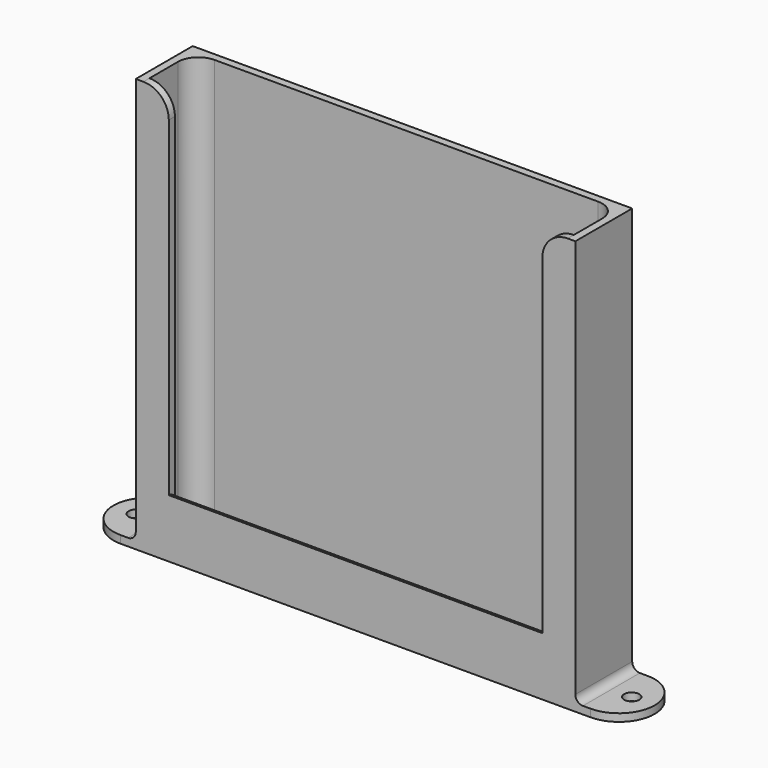
from build123d import *

# Parameters (mm, degrees)
F1_R     = 1.5
F2_DEPTH = 1.5
F3_DEPTH = 10
F4_DEPTH = 80
F5_R     = 5
F6_R     = 1.49999
F7_R     = 4


# Not quite as in the source:
# - a fillet or chamfer is up to 0.001 mm smaller than in the source, because OpenCascade refuses the exact size
# - a feature names something its author has since deleted; it is built from what else it names


with BuildPart() as f2:
    # F1 (on Top) → F2 (new body)
    with BuildSketch(Plane.XY):
        Polygon((-85, -12.5), (-85, -1.5), (-1.5, -1.5), (-1.5, -12.5), (0, -12.5), (0, 0), (-86.5, 0), (-86.5, -12.5), align=None)
        Polygon((-48.25, -12.5), (-80, -12.5), (-80, -14), (-6.5, -14), (-6.5, -12.5), (-38.25, -12.5), align=None)
        with BuildLine():
            Line((-1.5, -1.5), (-85, -1.5))
            Line((-85, -1.5), (-85, -12.5))
            Line((-85, -12.5), (-80, -12.5))
            Line((-80, -12.5), (-48.25, -12.5))
            ThreePointArc((-48.25, -12.5), (-49.6642135624, -11.9142135624), (-50.25, -10.5))
            Line((-50.25, -10.5), (-50.25, -7.5))
            ThreePointArc((-50.25, -7.5), (-49.6642135624, -6.0857864376), (-48.25, -5.5))
            Line((-48.25, -5.5), (-38.25, -5.5))
            ThreePointArc((-38.25, -5.5), (-36.8357864376, -6.0857864376), (-36.25, -7.5))
            Line((-36.25, -7.5), (-36.25, -10.5))
            ThreePointArc((-36.25, -10.5), (-36.8357864376, -11.9142135624), (-38.25, -12.5))
            Line((-38.25, -12.5), (-6.5, -12.5))
            Line((-6.5, -12.5), (-1.5, -12.5))
            Line((-1.5, -12.5), (-1.5, -1.5))
        make_face()
        with BuildLine():
            Line((-86.5, -14), (-86.5, -12.5))
            Line((-86.5, -12.5), (-86.5, 0))
            Line((-86.5, 0), (-89.5, 0))
            ThreePointArc((-89.5, 0), (-96.5, -7), (-89.5, -14))
            Line((-89.5, -14), (-86.5, -14))
        make_face()
        with Locations((-92, -7)):
            Circle(F1_R, mode=Mode.SUBTRACT)
        with BuildLine():
            Line((0, 0), (0, -12.5))
            Line((0, -12.5), (0, -14))
            Line((0, -14), (3, -14))
            ThreePointArc((3, -14), (10, -7), (3, 0))
            Line((3, 0), (0, 0))
        make_face()
        with Locations((5.5, -7)):
            Circle(F1_R, mode=Mode.SUBTRACT)
        Polygon((-80, -12.5), (-85, -12.5), (-86.5, -12.5), (-86.5, -14), (-80, -14), align=None)
        Polygon((0, -12.5), (-1.5, -12.5), (-6.5, -12.5), (-6.5, -14), (0, -14), align=None)
    extrude(amount=-F2_DEPTH)

    # F1 (on Top) → F3 (join)
    with BuildSketch(Plane.XY):
        Polygon((0, -12.5), (-1.5, -12.5), (-6.5, -12.5), (-6.5, -14), (0, -14), align=None)
        Polygon((-80, -12.5), (-85, -12.5), (-86.5, -12.5), (-86.5, -14), (-80, -14), align=None)
        Polygon((-48.25, -12.5), (-80, -12.5), (-80, -14), (-6.5, -14), (-6.5, -12.5), (-38.25, -12.5), align=None)
    extrude(amount=F3_DEPTH)

    # F1 (on Top) → F4 (join)
    with BuildSketch(Plane.XY):
        Polygon((-85, -12.5), (-85, -1.5), (-1.5, -1.5), (-1.5, -12.5), (0, -12.5), (0, 0), (-86.5, 0), (-86.5, -12.5), align=None)
        Polygon((-80, -12.5), (-85, -12.5), (-86.5, -12.5), (-86.5, -14), (-80, -14), align=None)
        Polygon((0, -12.5), (-1.5, -12.5), (-6.5, -12.5), (-6.5, -14), (0, -14), align=None)
    extrude(amount=F4_DEPTH)

    # F5
    f5_edges = [f2.edges().sort_by_distance(p)[0] for p in [
        (-80, -13.25, 80),
        (-6.5, -13.25, 80),
    ]]
    fillet(f5_edges, radius=F5_R)

    # F6 (radius 1.5 in the source; OpenCascade refuses exactly that, so slightly less here)
    f6_edges = [f2.edges().sort_by_distance(p)[0] for p in [
        (-43.25, -12.5, 10),
        (-86.5, -7, 0),
        (0, -7, 0),
    ]]
    fillet(f6_edges, radius=F6_R)

    # F7
    f7_edges = [f2.edges().sort_by_distance(p)[0] for p in [
        (-85, -1.5, 40),
        (-1.5, -1.5, 40),
    ]]
    fillet(f7_edges, radius=F7_R)


solid = f2.part
